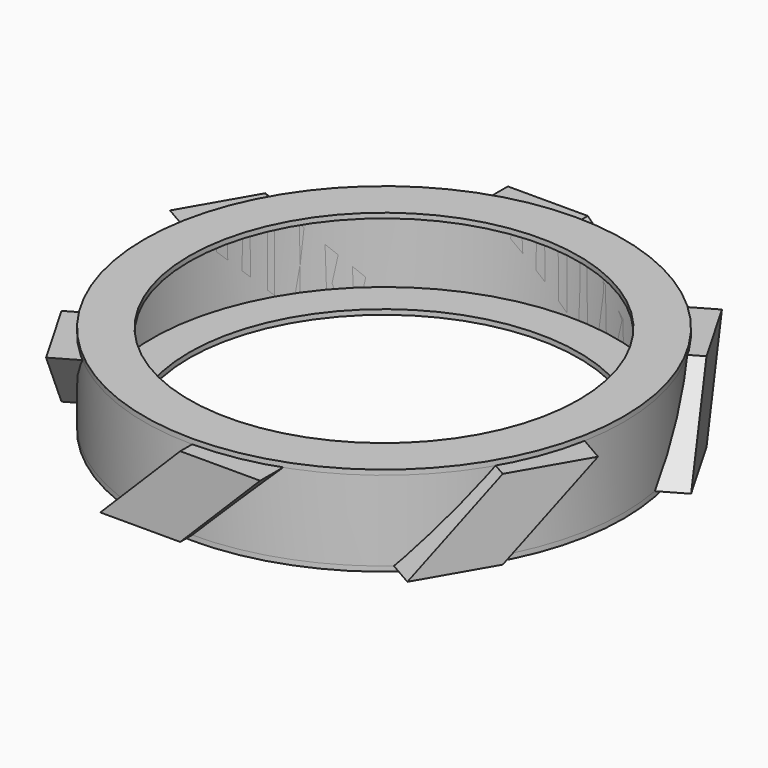
from build123d import *

# Parameters (mm, degrees)
F0_R     = 304.8
F0_R_2   = 295.275
F1_DEPTH = 101.6
F3_DEPTH = 323.85
F4_DEPTH = 254
F5_COUNT = 6
F6_DEPTH = 6.35
F7_R     = 304.8
F7_R_2   = 295.275
F7_R_3   = 247.65
F8_DEPTH = 6.35
F9_DEPTH = 127


# Not quite as in the source:
# - a feature names something its author has since deleted; it is built from what else it names


with BuildPart() as f1:
    # F0 (on Top) → F1 (new body)
    with BuildSketch(Plane.XY):
        Circle(F0_R)
        Circle(F0_R_2, mode=Mode.SUBTRACT)
    extrude(amount=F1_DEPTH)


with BuildPart() as f3:
    # F2 (on Front) → F3 (new body)
    with BuildSketch(Plane.XZ):
        Polygon((0, 101.6), (0, 0), (101.6, 0), align=None)
        Polygon((-101.6, 101.6), (0, 0), (0, 101.6), align=None)
    extrude(amount=-F3_DEPTH)

    # F0 (on Top) → F4 (cut)
    with BuildSketch(Plane.XY):
        Circle(F0_R_2)
    extrude(amount=F4_DEPTH, mode=Mode.SUBTRACT)


with BuildPart() as f5_1:
    # F5: instance of F3
    add(f3.part.rotate(Axis((0, 0, 50.8), (0, 0, -1)), 1 * 360 / F5_COUNT))


with BuildPart() as f5_2:
    # F5: instance of F3
    add(f3.part.rotate(Axis((0, 0, 50.8), (0, 0, -1)), 2 * 360 / F5_COUNT))


with BuildPart() as f5_3:
    # F5: instance of F3
    add(f3.part.rotate(Axis((0, 0, 50.8), (0, 0, -1)), 3 * 360 / F5_COUNT))


with BuildPart() as f5_4:
    # F5: instance of F3
    add(f3.part.rotate(Axis((0, 0, 50.8), (0, 0, -1)), 4 * 360 / F5_COUNT))


with BuildPart() as f5_5:
    # F5: instance of F3
    add(f3.part.rotate(Axis((0, 0, 50.8), (0, 0, -1)), 5 * 360 / F5_COUNT))


with BuildPart() as f6:
    # F0 (on Top) → F6 (new body)
    with BuildSketch(Plane.XY):
        Circle(F0_R)
        Circle(F0_R_2, mode=Mode.SUBTRACT)
        Circle(F0_R_2)
    extrude(amount=-F6_DEPTH)

    # F7 (on face) → F9 (cut)
    with BuildSketch(Plane.XY.offset(101.6)):
        Circle(F7_R_3)
    extrude(amount=-F9_DEPTH, mode=Mode.SUBTRACT)


with BuildPart() as f8:
    # F7 (on face) → F8 (new body)
    with BuildSketch(Plane.XY.offset(101.6)):
        Circle(F7_R)
        Circle(F7_R_2, mode=Mode.SUBTRACT)
        Circle(F7_R_2)
        Circle(F7_R_3, mode=Mode.SUBTRACT)
    extrude(amount=F8_DEPTH)


solid = Compound([f1.part, f3.part, f5_1.part, f5_2.part, f5_3.part, f5_4.part, f5_5.part, f6.part, f8.part])
